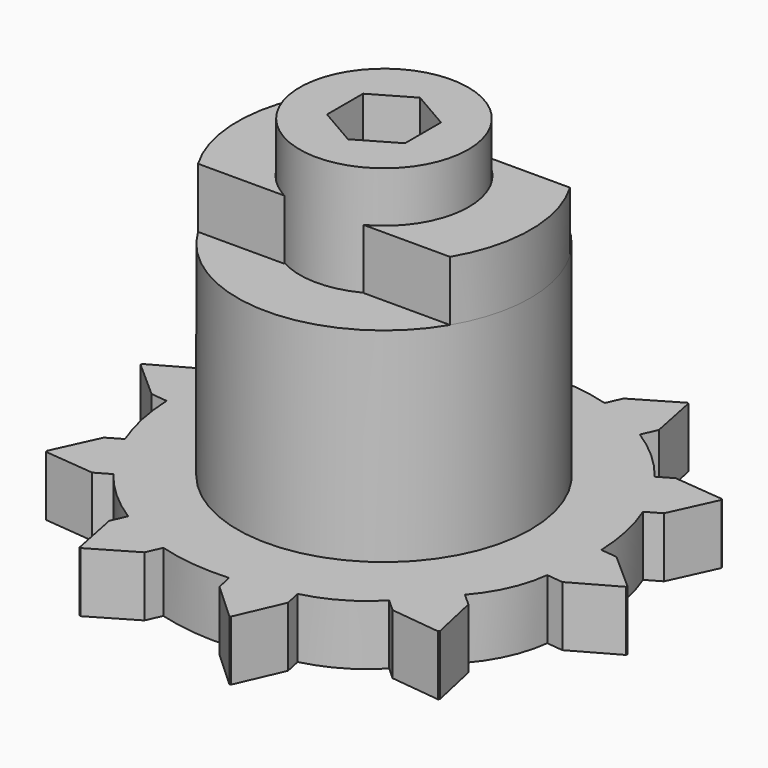
from build123d import *
from build123d import SkipClean  # not in build123d's __all__

# Parameters (mm, degrees)
F0_R           = 11.303
F0_R_2         = 5.715
F1_DEPTH       = 2.54
F5_R           = 3.5687
F6_DEPTH       = 4.6736
F6_DEPTH_BACK  = 5.08
F8_DEPTH       = 50.8
F10_DEPTH      = 25.4
F13_DEPTH      = 25.4
F4_R           = 6.2103
F15_DEPTH      = 11.176
F16_DEPTH      = 50.8
F16_DEPTH_BACK = 50.8
F18_DEPTH      = 2.54


with BuildPart() as f1:
    # F0 (on Top) → F1 (new body)
    with BuildSketch(Plane.XY):
        Circle(F0_R)
        Circle(F0_R_2, mode=Mode.SUBTRACT)
    extrude(amount=F1_DEPTH)

    # F9 (on face) → F10 (cut)
    with BuildSketch(Plane(origin=(0, 0, 0), x_dir=(1, 0, 0), z_dir=(0, 0, -1))):
        with BuildLine():
            Line((-8.9271557155, 3.6697404311), (-9.8146830534, 5.6062291749))
            ThreePointArc((-9.8146830534, 5.6062291749), (-11.0597926204, 2.3321226799), (-11.242701421, -1.1659647326))
            Line((-11.242701421, -1.1659647326), (-9.6488317662, 0.2472843445))
            Line((-9.6488317662, 0.2472843445), (-8.9477035333, 0.3221237808))
            ThreePointArc((-8.9477035333, 0.3221237808), (-8.7608469633, 1.847355606), (-8.3159415428, 3.3181739717))
            Line((-8.3159415428, 3.3181739717), (-8.9271557155, 3.6697404311))
        make_face()
        with BuildLine():
            Line((-4.7773643073, 7.5724469312), (-5.0652013801, 8.2161328482))
            Line((-5.0652013801, 8.2161328482), (-4.6449865546, 10.3044606316))
            ThreePointArc((-4.6449865546, 10.3044606316), (-7.5767728664, 8.3875098767), (-9.7808733868, 5.6650088077))
            Line((-9.7808733868, 5.6650088077), (-7.6607187839, 5.8714982512))
            Line((-7.6607187839, 5.8714982512), (-7.0495046113, 5.5199317918))
            ThreePointArc((-7.0495046113, 5.5199317918), (-6.0018256975, 6.6440387225), (-4.7773643073, 7.5724469312))
        make_face()
        with BuildLine():
            ThreePointArc((2.2989369307, 11.0667383627), (-1.1996834025, 11.2391533815), (-4.5830841585, 10.33214153))
            Line((-4.5830841585, 10.33214153), (-2.7464716044, 9.2529993908))
            Line((-2.7464716044, 9.2529993908), (-2.4586345316, 8.6093134738))
            ThreePointArc((-2.4586345316, 8.6093134738), (-0.9503110098, 8.9029248696), (0.586003717, 8.934302541))
            Line((0.586003717, 8.934302541), (0.7314877226, 9.6242417733))
            Line((0.7314877226, 9.6242417733), (2.2989369307, 11.0667383627))
        make_face()
        with BuildLine():
            ThreePointArc((8.3647446465, 7.6018981839), (5.6356443454, 9.7978222995), (2.3652874451, 11.0527473644))
            Line((2.3652874451, 11.0527473644), (3.2168343788, 9.100169261))
            Line((3.2168343788, 9.100169261), (3.0713503732, 8.4102300286))
            ThreePointArc((3.0713503732, 8.4102300286), (4.5083713952, 7.8380073479), (5.7255382389, 6.8835582459))
            Line((5.7255382389, 6.8835582459), (6.2487733776, 7.356217457))
            Line((6.2487733776, 7.356217457), (8.3647446465, 7.6018981839))
        make_face()
        with BuildLine():
            ThreePointArc((11.2355042146, 1.2333912778), (10.3183475019, 4.6140561147), (8.4101996378, 7.5515793747))
            Line((8.4101996378, 7.5515793747), (7.9514189656, 5.4713837769))
            Line((7.9514189656, 5.4713837769), (7.4281838269, 4.9987245658))
            ThreePointArc((7.4281838269, 4.9987245658), (8.2664076362, 3.6964900333), (8.6781117575, 2.2035286644))
            Line((8.6781117575, 2.2035286644), (9.3792399904, 2.2783681008))
            Line((9.3792399904, 2.2783681008), (11.2355042146, 1.2333912778))
        make_face()
        with BuildLine():
            ThreePointArc((11.303, 0), (11.2879152894, 0.5837614402), (11.242701421, 1.1659647326))
            Line((11.242701421, 1.1659647326), (9.6488317662, -0.2472843445))
            Line((9.6488317662, -0.2472843445), (8.9477035333, -0.3221237809))
            ThreePointArc((8.9477035333, -0.3221237808), (8.7608469633, -1.847355606), (8.3159415428, -3.3181739717))
            Line((8.3159415428, -3.3181739717), (8.9271557155, -3.6697404311))
            Line((8.9271557155, -3.6697404311), (9.8146830534, -5.6062291749))
            ThreePointArc((9.8146830534, -5.6062291749), (10.9245862977, -2.900210893), (11.303, 0))
        make_face()
        with BuildLine():
            ThreePointArc((4.6449865546, -10.3044606316), (7.5767728664, -8.3875098767), (9.7808733868, -5.6650088077))
            Line((9.7808733868, -5.6650088077), (7.6607187839, -5.8714982512))
            Line((7.6607187839, -5.8714982512), (7.0495046113, -5.5199317918))
            ThreePointArc((7.0495046113, -5.5199317918), (6.0018256975, -6.6440387225), (4.7773643073, -7.5724469312))
            Line((4.7773643073, -7.5724469312), (5.0652013801, -8.2161328482))
            Line((5.0652013801, -8.2161328482), (4.6449865546, -10.3044606316))
        make_face()
        with BuildLine():
            Line((-0.7314877226, -9.6242417733), (-2.2989369307, -11.0667383627))
            ThreePointArc((-2.2989369307, -11.0667383627), (1.1996834025, -11.2391533815), (4.5830841585, -10.33214153))
            Line((4.5830841585, -10.33214153), (2.7464716044, -9.2529993908))
            Line((2.7464716044, -9.2529993908), (2.4586345316, -8.6093134738))
            ThreePointArc((2.4586345316, -8.6093134738), (0.9503110098, -8.9029248696), (-0.586003717, -8.934302541))
            Line((-0.586003717, -8.934302541), (-0.7314877226, -9.6242417733))
        make_face()
        with BuildLine():
            Line((-6.2487733776, -7.356217457), (-8.3647446465, -7.6018981839))
            ThreePointArc((-8.3647446465, -7.6018981839), (-5.6356443454, -9.7978222995), (-2.3652874451, -11.0527473644))
            Line((-2.3652874451, -11.0527473644), (-3.2168343788, -9.100169261))
            Line((-3.2168343788, -9.100169261), (-3.0713503732, -8.4102300286))
            ThreePointArc((-3.0713503732, -8.4102300286), (-4.4641901838, -7.7611963159), (-5.7255382389, -6.8835582459))
            Line((-5.7255382389, -6.8835582459), (-6.2487733776, -7.356217457))
        make_face()
        with BuildLine():
            Line((-9.3792399904, -2.2783681008), (-11.2355042146, -1.2333912778))
            ThreePointArc((-11.2355042146, -1.2333912778), (-10.3183475019, -4.6140561147), (-8.4101996378, -7.5515793747))
            Line((-8.4101996378, -7.5515793747), (-7.9514189656, -5.4713837769))
            Line((-7.9514189656, -5.4713837769), (-7.4281838269, -4.9987245658))
            ThreePointArc((-7.4281838269, -4.9987245658), (-8.1735224594, -3.6549545628), (-8.6781117575, -2.2035286644))
            Line((-8.6781117575, -2.2035286644), (-9.3792399904, -2.2783681008))
        make_face()
    extrude(amount=-F10_DEPTH, mode=Mode.SUBTRACT)


with BuildPart() as f6:
    # F5 (on offset) → F6 (new body, two sides)
    with BuildSketch(Plane.XY.offset(11.176)) as f6_sk:
        Circle(F5_R)
    extrude(amount=F6_DEPTH)
    extrude(f6_sk.sketch, amount=-F6_DEPTH_BACK)

    # F7 (on offset) → F8 (cut)
    with BuildSketch(Plane.XY.offset(11.176)):
        Polygon((1.5165992773, 0.4486275472), (0.369776786, 1.5377272751), (-1.1468224914, 1.089099728), (-1.5165992773, -0.4486275472), (-0.369776786, -1.5377272751), (1.1468224914, -1.089099728), align=None)
    extrude(amount=-F8_DEPTH, mode=Mode.SUBTRACT)

    # F12 (on face) → F13 (cut)
    with BuildSketch(Plane.XY.offset(15.8496)):
        Polygon((0, 1.9064105889), (-1.651, 0.9532052944), (-1.651, -0.9532052944), (0, -1.9064105889), (1.651, -0.9532052944), (1.651, 0.9532052944), align=None)
    extrude(amount=-F13_DEPTH, mode=Mode.SUBTRACT)


with BuildPart() as f15:
    # F4 (on offset) → F15 (new body, through all)
    with BuildSketch(Plane.XY.offset(11.176)):
        Circle(F4_R)
    extrude(amount=-F15_DEPTH)

    # F14 (on face) → F16 (cut, two sides)
    with BuildSketch(Plane.XY.offset(2.54)) as f16_sk:
        Polygon((0, 1.9064105889), (-1.651, 0.9532052944), (-1.651, -0.9532052944), (0, -1.9064105889), (1.651, -0.9532052944), (1.651, 0.9532052944), align=None)
    extrude(amount=-F16_DEPTH, mode=Mode.SUBTRACT)
    extrude(f16_sk.sketch, amount=F16_DEPTH_BACK, mode=Mode.SUBTRACT)

    # F17 (on face) → F18 (join)
    with BuildSketch(Plane.XY.offset(11.176)):
        with BuildLine():
            ThreePointArc((-1.6756872114, -3.175), (-1.7915606918, -3.1110870959), (-1.905, -3.0429471948))
            ThreePointArc((-1.905, -3.0429471948), (-3.5900630399, 0), (-1.905, 3.0429471948))
            ThreePointArc((-1.905, 3.0429471948), (-1.7915606918, 3.1110870959), (-1.6756872114, 3.175))
            Line((-1.6756872114, 3.175), (-5.3373402637, 3.175))
            ThreePointArc((-5.3373402637, 3.175), (-6.2103, 0), (-5.3373402637, -3.175))
            Line((-5.3373402637, -3.175), (-1.6756872114, -3.175))
        make_face()
        with BuildLine():
            ThreePointArc((1.6756872114, 3.175), (2.7219479771, 2.340844258), (3.3900758016, 1.1814984934))
            ThreePointArc((3.3900758016, 1.1814984934), (3.5900630399, 0), (3.3900758016, -1.1814984934))
            ThreePointArc((3.3900758016, -1.1814984934), (2.7219479771, -2.340844258), (1.6756872114, -3.175))
            Line((1.6756872114, -3.175), (5.3373402637, -3.175))
            ThreePointArc((5.3373402637, -3.175), (6.2103, 0), (5.3373402637, 3.175))
            Line((5.3373402637, 3.175), (1.6756872114, 3.175))
        make_face()
    with SkipClean():  # cleaning this boolean's faces spoils the solid; the shape is the same uncleaned
        extrude(amount=F18_DEPTH)


solid = Compound([f1.part, f6.part, f15.part])
